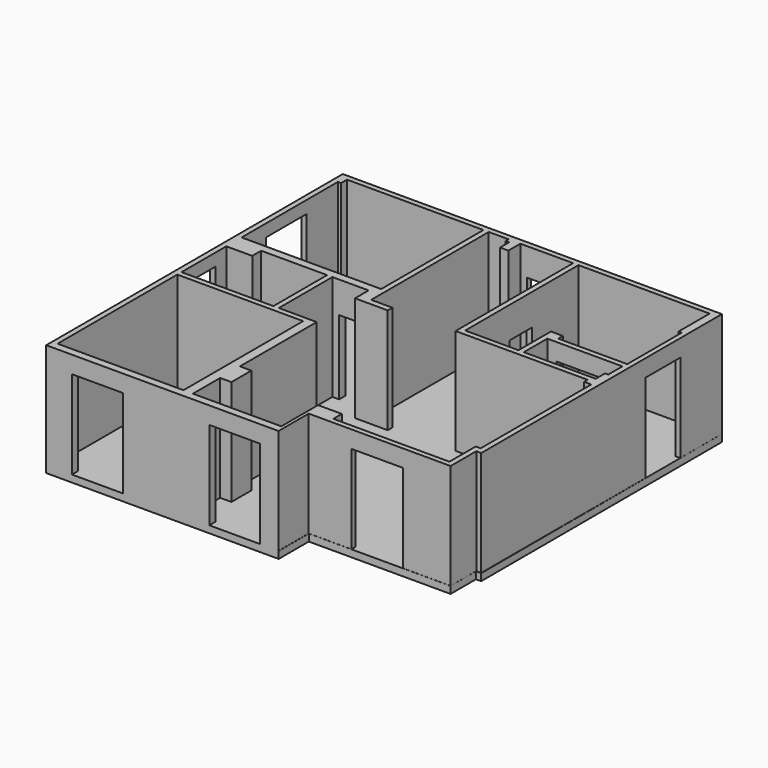
from build123d import *

# Parameters (mm, degrees)
F0_W      = 3562
F0_H      = 4233.004609108
F1_DEPTH  = 2985
F2_W      = 1450
F2_H      = 2500
F3_DEPTH  = 144.9
F4_W      = 1440
F4_H      = 2500
F5_DEPTH  = 213.304599762
F6_W      = 1443
F6_H      = 2500
F7_DEPTH  = 213.304599762
F8_W      = 797
F8_H      = 2500
F9_DEPTH  = 4156.8055872194
F10_W     = 800
F10_H     = 2100
F11_DEPTH = 150
F12_W     = 1042
F12_H     = 2200
F13_DEPTH = 150
F14_W     = 1235
F14_H     = 2500
F15_DEPTH = 137.5694923401
F16_W     = 700
F16_H     = 2100
F17_DEPTH = 153.3939067339
F18_W     = 794
F18_H     = 2100
F19_DEPTH = 225.0975813866
F20_W     = 646
F20_H     = 2100
F21_DEPTH = 150
F22_W     = 640
F22_H     = 1550
F23_DEPTH = 150
F24_W     = 1438
F24_H     = 1550
F25_DEPTH = 150
F27_DEPTH = 200
F28_W     = 1800
F28_H     = 2500
F29_DEPTH = 150


with BuildPart() as f1:
    # F0 (on Top) → F1 (new body)
    with BuildSketch(Plane.XY):
        Polygon((1409, -5111.9), (2800.470790863, -5111.9), (4212.9532585144, -5111.9), (4212.9532585144, -4204.4310569763), (4352.9532585144, -4204.4310569763), (4352.9532585144, 4306.8055872194), (-2273.6162338257, 4306.8055872194), (-6372.8999999957, 4306.8055872194), (-6372.8999999957, 541.0975813866), (-6372.8999999957, -6179.304599762), (-2660.8999999957, -6179.304599762), (-1872.0002385101, -6179.304599762), (-435.1912385101, -6179.304599762), (198.84583354, -6179.304599762), (198.84583354, -5111.9), (720.84583354, -5111.9), (1350.470790863, -5111.9), align=None)
        with Locations((-4441.8999999957, -3849.497695446)):
            Rectangle(F0_W, F0_H, mode=Mode.SUBTRACT)
        Polygon((-5487.8999999957, 316), (-3622.8999999957, 316), (-3622.8999999957, -1583), (-6222.8999999957, -1583), (-6222.8999999957, 0), (-5487.8999999957, 0), align=None, mode=Mode.SUBTRACT)
        Polygon((-6132.8999999957, 4156.8055872194), (-2273.6162338257, 4156.8055872194), (-2273.6162338257, 541.0975813866), (-3622.8999999957, 541.0975813866), (-6222.8999999957, 541.0975813866), (-6222.8999999957, 3944.8055872194), (-6132.8999999957, 3944.8055872194), align=None, mode=Mode.SUBTRACT)
        Polygon((264.3837661743, 4156.8055872194), (264.3837661743, 0), (4001, 0), (4001, -125), (4202.9532585144, -125), (4202.9532585144, -4036), (4062.9532585144, -4036), (4062.9532585144, -4501.5), (4062.9532585144, -4967), (2970.9532585144, -4967), (1520.9532585144, -4967), (778.9532585144, -4967), (778.9532585144, -4667), (106.9532585144, -4667), (106.9532585144, -5966), (-320.0467414856, -5966), (-1760.0467414856, -5966), (-2394.0467414856, -5966), (-2394.0467414856, -5002), (-2075.0467414856, -5002), (-2075.0467414856, -4297), (-2399.0467414856, -4297), (-2399.0467414856, -1583), (-2660.8999999957, -1583), (-3472.8999999957, -1579.3216228485), (-3472.8999999957, 316), (-2448.6162338257, 316), (-2448.6162338257, -166), (-2123.6162338257, -166), (-1523.6162338257, -166), (-1523.6162338257, 0), (-2123.6162338257, 0), (-2123.6162338257, 150), (-2123.6162338257, 4156.8055872194), (-1562.6162338257, 4156.8055872194), (-1562.6162338257, 4055.8055872194), (-1461.6162338257, 4055.8055872194), (-1461.6162338257, 3731.8055872194), (-1227.6162338257, 3731.8055872194), (-1227.6162338257, 4156.8055872194), align=None, mode=Mode.SUBTRACT)
        Polygon((4198.8945047255, 981.3654631398), (4198.8945047255, 479.3654631398), (4108.8945047255, 479.3654631398), (4108.8945047255, 149.4008999277), (2259.8945047255, 149.7780185152), (2073.5213682051, 149.8160308321), (2073.5213682051, 981.3654631398), align=None, mode=Mode.SUBTRACT)
        Polygon((4215.3837661743, 1131.3654631398), (2262.5213682051, 1131.3654631398), (2262.5213682051, 1296.3654631398), (1923.5213682051, 1296.3654631398), (1923.5213682051, 150), (414.3837661743, 150), (414.3837661743, 1131.3654631398), (414.3837661743, 4156.8055872194), (4125.3837661743, 4156.8055872194), (4125.3837661743, 3063.8055872194), (4215.3837661743, 3063.8055872194), align=None, mode=Mode.SUBTRACT)
    extrude(amount=F1_DEPTH)

    # F2 (on face) → F3 (cut, through all)
    with BuildSketch(Plane.XZ.offset(5111.9)):
        with Locations((2134, 1250)):
            Rectangle(F2_W, F2_H)
    extrude(amount=-F3_DEPTH, mode=Mode.SUBTRACT)

    # F4 (on face) → F5 (cut, through all)
    with BuildSketch(Plane.XZ.offset(6179.304599762)):
        with Locations((-1040.0467414856, 1250)):
            Rectangle(F4_W, F4_H)
    extrude(amount=-F5_DEPTH, mode=Mode.SUBTRACT)

    # F6 (on face) → F7 (cut, through all)
    with BuildSketch(Plane.XZ.offset(6179.304599762)):
        with Locations((-4923.3999999957, 1250)):
            Rectangle(F6_W, F6_H)
    extrude(amount=-F7_DEPTH, mode=Mode.SUBTRACT)

    # F8 (on face) → F9 (cut, through all)
    with BuildSketch(Plane.XZ):
        with Locations((-398.5, 1250)):
            Rectangle(F8_W, F8_H)
    extrude(amount=-F9_DEPTH, mode=Mode.SUBTRACT)

    # F10 (on face) → F11 (cut, through all)
    with BuildSketch(Plane(origin=(264.3837661743, 0, 0), x_dir=(0, -1, 0), z_dir=(-1, 0, 0))):
        with Locations((-2115.4956257177, 1050)):
            Rectangle(F10_W, F10_H)
    extrude(amount=-F11_DEPTH, mode=Mode.SUBTRACT)

    # F12 (on face) → F13 (cut, through all)
    with BuildSketch(Plane.XZ.offset(-4156.8055872194)):
        with Locations((-521, 1100)):
            Rectangle(F12_W, F12_H)
    extrude(amount=-F13_DEPTH, mode=Mode.SUBTRACT)

    # F14 (on face) → F15 (cut, through all)
    with BuildSketch(Plane(origin=(4215.3837661743, 0, 0), x_dir=(0, -1, 0), z_dir=(-1, 0, 0))):
        with Locations((-2216.3055872194, 1250)):
            Rectangle(F14_W, F14_H)
    extrude(amount=-F15_DEPTH, mode=Mode.SUBTRACT)

    # F16 (on face) → F17 (cut, through all)
    with BuildSketch(Plane.XZ.offset(1732.995390892)):
        with Locations((-3060.8999999957, 1050)):
            Rectangle(F16_W, F16_H)
    extrude(amount=-F17_DEPTH, mode=Mode.SUBTRACT)

    # F18 (on face) → F19 (cut, through all)
    with BuildSketch(Plane.XZ.offset(-316)):
        with Locations((-2885.8999999957, 1050)):
            Rectangle(F18_W, F18_H)
    extrude(amount=-F19_DEPTH, mode=Mode.SUBTRACT)

    # F20 (on face) → F21 (cut, through all)
    with BuildSketch(Plane.YZ.offset(-3472.8999999957)):
        with Locations((-716, 1050)):
            Rectangle(F20_W, F20_H)
    extrude(amount=-F21_DEPTH, mode=Mode.SUBTRACT)

    # F22 (on face) → F23 (cut, through all)
    with BuildSketch(Plane.YZ.offset(-6222.8999999957)):
        with Locations((-707.1478068829, 1860)):
            Rectangle(F22_W, F22_H)
    extrude(amount=-F23_DEPTH, mode=Mode.SUBTRACT)

    # F24 (on face) → F25 (cut, through all)
    with BuildSketch(Plane.YZ.offset(-6222.8999999957)):
        with Locations((2119.8055872194, 1860)):
            Rectangle(F24_W, F24_H)
    extrude(amount=-F25_DEPTH, mode=Mode.SUBTRACT)

    # F26 (on face) → F27 (join)
    with BuildSketch(Plane(origin=(0, 0, 0), x_dir=(1, 0, 0), z_dir=(0, 0, -1))):
        Polygon((202.7448713779, 6179.304599762), (-6377.0327568054, 6179.304599762), (-6373.4097480774, -4305.7265281677), (4353.7154197693, -4305.7265281677), (4361.6199493408, 4216.0544395447), (4213.9821052551, 4216.0544395447), (4213.9821052551, 5115.1938438416), (202.7448713779, 5115.1938438416), align=None)
    extrude(amount=F27_DEPTH)

    # F28 (on face) → F29 (cut, through all)
    with BuildSketch(Plane(origin=(0, 1131.3654631398, 0), x_dir=(-1, 0, 0), z_dir=(0, 1, 0))):
        with Locations((-3232.5213682051, 1250)):
            Rectangle(F28_W, F28_H)
    extrude(amount=-F29_DEPTH, mode=Mode.SUBTRACT)


solid = f1.part
